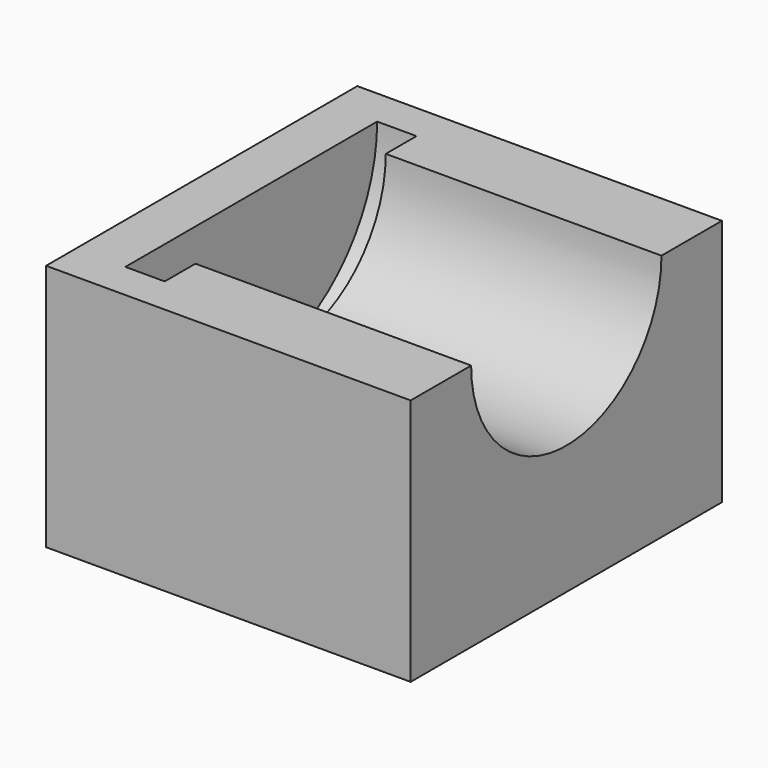
from build123d import *

# Parameters (mm, degrees)
F1_DEPTH  = 145
F2_W      = 15.7
F2_H      = 15
F3_DEPTH  = 11.463
F4_W      = 15.7
F4_H      = 15
F5_DEPTH  = 11.463
F7_DEPTH  = 25.427
F8_R      = 6.35
F8_R_2    = 4.8005
F9_DEPTH  = 1.5875
F10_R     = 6.35
F11_DEPTH = 1.5875
F12_W     = 129.3
F12_H     = 2.5
F12_H_2   = 15
F13_DEPTH = 25.427
F15_DEPTH = 25.427
F16_W     = 12.713
F16_H     = 10
F17_DEPTH = 15.701
F19_DEPTH = 2


with BuildPart() as f1:
    # F0 (on Front) → F1 (new body)
    with BuildSketch(Plane.XZ):
        Polygon((0, 2.5), (0, 0), (12.713, 0), (25.426, 0), (25.426, 2.5), (13.963, 2.5), (13.963, 17.5), (25.426, 17.5), (25.426, 20), (12.713, 20), (0, 20), (0, 17.5), (11.463, 17.5), (11.463, 2.5), align=None)
    extrude(amount=-F1_DEPTH)

    # F2 (on face) → F3 (join, through all)
    with BuildSketch(Plane.YZ.offset(13.963)):
        with Locations((7.85, 10)):
            Rectangle(F2_W, F2_H)
    extrude(amount=F3_DEPTH)

    # F4 (on face) → F5 (join, through all)
    with BuildSketch(Plane(origin=(11.463, 0, 0), x_dir=(0, -1, 0), z_dir=(-1, 0, 0))):
        with Locations((-7.85, 10)):
            Rectangle(F4_W, F4_H)
    extrude(amount=F5_DEPTH)

    # F6 (on face) → F7 (cut, through all)
    with BuildSketch(Plane.YZ.offset(25.426)):
        with BuildLine():
            Line((3.0495, 10), (12.6505, 10))
            ThreePointArc((12.6505, 10), (7.85, 14.8005), (3.0495, 10))
        make_face()
        with BuildLine():
            ThreePointArc((3.0495, 10), (7.85, 5.1995), (12.6505, 10))
            Line((12.6505, 10), (3.0495, 10))
        make_face()
    extrude(amount=-F7_DEPTH, mode=Mode.SUBTRACT)

    # F8 (on face) → F9 (cut)
    with BuildSketch(Plane.YZ.offset(25.426)):
        with Locations((7.85, 10)):
            Circle(F8_R)
        with Locations((7.85, 10)):
            Circle(F8_R_2, mode=Mode.SUBTRACT)
    extrude(amount=-F9_DEPTH, mode=Mode.SUBTRACT)

    # F10 (on face) → F11 (cut)
    with BuildSketch(Plane(origin=(0, 0, 0), x_dir=(0, -1, 0), z_dir=(-1, 0, 0))):
        with Locations((-7.85, 10)):
            Circle(F10_R)
    extrude(amount=-F11_DEPTH, mode=Mode.SUBTRACT)

    # F12 (on face) → F13 (cut, through all)
    with BuildSketch(Plane.YZ.offset(25.426)):
        with Locations((80.35, 18.75)):
            Rectangle(F12_W, F12_H)
        with Locations((80.35, 10)):
            Rectangle(F12_W, F12_H_2)
        with Locations((80.35, 1.25)):
            Rectangle(F12_W, F12_H)
    extrude(amount=-F13_DEPTH, mode=Mode.SUBTRACT)

    # F14 (on face) → F15 (cut, through all)
    with BuildSketch(Plane(origin=(0, 0, 0), x_dir=(0, -1, 0), z_dir=(-1, 0, 0))):
        with BuildLine():
            ThreePointArc((-14.2, 10), (-7.85, 16.35), (-1.5, 10))
            Line((-1.5, 10), (0, 10))
            Line((0, 10), (0, 20))
            Line((0, 20), (-15.7, 20))
            Line((-15.7, 20), (-15.7, 10))
            Line((-15.7, 10), (-14.2, 10))
        make_face()
        with BuildLine():
            Line((-14.2, 10), (-1.5, 10))
            ThreePointArc((-1.5, 10), (-7.85, 16.35), (-14.2, 10))
        make_face()
    extrude(amount=-F15_DEPTH, mode=Mode.SUBTRACT)

    # F16 (on face) → F17 (cut, through all)
    with BuildSketch(Plane.XZ):
        with Locations((19.0695, 5)):
            Rectangle(F16_W, F16_H)
    extrude(amount=-F17_DEPTH, mode=Mode.SUBTRACT)

    # F18 (on face) → F19 (join)
    with BuildSketch(Plane(origin=(0, 0, 0), x_dir=(0, -1, 0), z_dir=(-1, 0, 0))):
        with BuildLine():
            Line((-14.2, 10), (-15.7, 10))
            Line((-15.7, 10), (-15.7, 0))
            Line((-15.7, 0), (0, 0))
            Line((0, 0), (0, 10))
            Line((0, 10), (-1.5, 10))
            ThreePointArc((-1.5, 10), (-7.85, 3.65), (-14.2, 10))
        make_face()
        with BuildLine():
            Line((-1.5, 10), (-14.2, 10))
            ThreePointArc((-14.2, 10), (-7.85, 3.65), (-1.5, 10))
        make_face()
    extrude(amount=F19_DEPTH)


solid = f1.part
